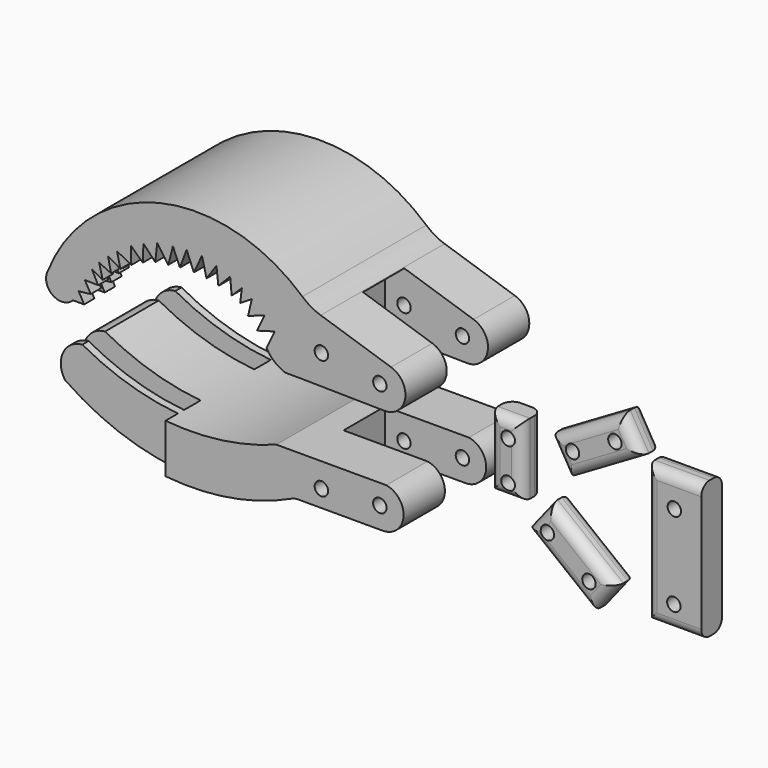
from build123d import *

# Parameters (mm, degrees)
F2_DEPTH       = 38.1
F3_DEPTH       = 38.1
F1_W           = 6.35
F1_H           = 59.9533222238
F4_DEPTH       = 50.8
F1_W_2         = 38.1
F7_DEPTH       = 101.6
F11_D          = 6.604
F11_2_D        = 6.604
F12_W          = 25.4
F12_H          = 93.7925264519
F13_DEPTH      = 25.4
F16_D          = 6.604
F16_DEPTH      = 38.101
F16_2_D        = 6.604
F16_2_DEPTH    = 38.101
F17_D          = 6.604
F17_2_D        = 6.604
F18_W          = 7.62
F18_H          = 40.64
F19_DEPTH      = 76.2
F18_W_2        = 10.16
F0_W           = 15.8650130033
F0_H           = 34.8350182176
F22_DEPTH      = 12.7
F0_W_2         = 26.9726514816
F0_H_2         = 67.5600729883
F23_D          = 6.604
F23_2_D        = 6.604
F23_3_D        = 6.604
F23_4_D        = 6.604
F24_T1_DEPTH   = 60.2350182176
F24_T3_DEPTH   = 41.2650130033
F24_2_T1_DEPTH = 43.5777924299
F24_2_T3_DEPTH = 43.5777924299
F24_2_T5_DEPTH = 66.6787329406
F24_2_T7_DEPTH = 66.6787329406
F24_3_T1_DEPTH = 52.3726514816
F24_3_T3_DEPTH = 92.9600729883
F24_4_T1_DEPTH = 66.6787329406
F24_4_T3_DEPTH = 66.6787329406
F24_4_T5_DEPTH = 43.5777924299
F24_4_T7_DEPTH = 43.5777924299


# Not quite as in the source:
# - a fillet or chamfer that OpenCascade refuses, or shapes differently, is made with other operations: its cross-section is extruded or revolved along the edge and cut away or added


with BuildPart() as f2:
    # F0 (on Front) → F2 (new body, symmetric)
    with BuildSketch(Plane.XZ):
        with BuildLine():
            ThreePointArc((-128.8251806366, 24.5439261482), (-120.2352063415, 28.3244505451), (-114.4677234787, 20.9206566167))
            ThreePointArc((-114.4677234787, 20.9206566167), (-115.0121445518, 18.0890647902), (-116.567776135, 15.6612433482))
            Line((-116.567776135, 15.6612433482), (-111.0370755196, 15.6612433482))
            Line((-111.0370755196, 15.6612433482), (-113.6851459746, 20.5360539255))
            Line((-113.6851459746, 20.5360539255), (-107.745103538, 21.214004606))
            Line((-107.745103538, 21.214004606), (-110.6837838888, 26.4116507024))
            Line((-110.6837838888, 26.4116507024), (-104.1332259774, 26.230096817))
            Line((-104.1332259774, 26.230096817), (-107.1282997727, 32.1294739842))
            Line((-107.1282997727, 32.1294739842), (-101.9096150994, 29.2251650244))
            Line((-101.9096150994, 29.2251650244), (-103.6340519786, 36.2136624753))
            Line((-103.6340519786, 36.2136624753), (-97.7411866188, 33.430468291))
            Line((-97.7411866188, 33.430468291), (-99.2413535714, 40.3858050704))
            Line((-99.2413535714, 40.3858050704), (-93.1724831462, 36.8399471045))
            Line((-93.1724831462, 36.8399471045), (-94.8431268334, 44.0680421889))
            Line((-94.8431268334, 44.0680421889), (-87.853692472, 40.2494259179))
            Line((-87.853692472, 40.2494259179), (-87.853692472, 48.4662689269))
            Line((-87.853692472, 48.4662689269), (-82.1257680654, 43.1474819779))
            Line((-82.1257680654, 43.1474819779), (-81.8530097604, 51.6029894352))
            Line((-81.8530097604, 51.6029894352), (-76.0227963328, 45.3636422753))
            Line((-76.0227963328, 45.3636422753), (-75.0340521335, 53.9896264672))
            Line((-75.0340521335, 53.9896264672), (-69.6129798889, 46.2842024863))
            Line((-69.6129798889, 46.2842024863), (-67.3286244273, 55.1488474011))
            Line((-67.3286244273, 55.1488474011), (-63.8850554824, 46.9320043921))
            Line((-63.8850554824, 46.9320043921), (-60.5778545141, 55.8307431638))
            Line((-60.5778545141, 55.8307431638), (-57.0319965482, 47.0683835447))
            Line((-57.0319965482, 47.0683835447), (-53.008813411, 55.6943640113))
            Line((-53.008813411, 55.6943640113), (-50.7926493883, 46.5228669345))
            Line((-50.7926493883, 46.5228669345), (-45.9170974791, 53.6486767232))
            Line((-45.9170974791, 53.6486767232), (-44.9624434113, 45.1590754092))
            Line((-44.9624434113, 45.1590754092), (-39.1663275659, 51.1597581208))
            Line((-39.1663275659, 51.1597581208), (-38.4162440896, 43.1474819779))
            Line((-38.4162440896, 43.1474819779), (-33.4043093026, 47.9889400303))
            Line((-33.4043093026, 47.9889400303), (-34.2225842178, 41.2722676992))
            Line((-34.2225842178, 41.2722676992), (-28.4946598112, 44.8181256652))
            Line((-28.4946598112, 44.8181256652), (-30.3357802331, 36.9081310928))
            Line((-30.3357802331, 36.9081310928), (-22.2009439021, 39.8494154215))
            Line((-22.2009439021, 39.8494154215), (-26.0398332029, 31.9643877447))
            Line((-26.0398332029, 31.9643877447), (-17.2234997153, 34.4656482339))
            Line((-17.2234997153, 34.4656482339), (-21.2665628641, 25.99779889))
            ThreePointArc((-21.2665628641, 25.99779889), (-17.3327439292, 21.2846448873), (-11.9722324247, 18.2923767716))
            Line((-11.9722324247, 18.2923767716), (-5.0168965772, 18.2923767716))
            Line((-5.0168965772, 18.2923767716), (36.7117887588, 17.6685203985))
            ThreePointArc((36.7117887588, 17.6685203985), (26.7700458222, 29.5718005255), (40.0189591139, 37.6336010062))
            Line((40.0189591139, 37.6336010062), (5.4235169889, 48.8439725139))
            ThreePointArc((5.4235169889, 48.8439725139), (0.643395485, 50.9582523352), (-3.6027484392, 54.0062028812))
            ThreePointArc((-3.6027484392, 54.0062028812), (-73.8525944836, 71.7412526891), (-128.8251806366, 24.5439261482))
        make_face()
        with BuildLine():
            ThreePointArc((-116.567776135, 15.6612433482), (-115.0121445518, 18.0890647902), (-114.4677234787, 20.9206566167))
            ThreePointArc((-114.4677234787, 20.9206566167), (-120.2352063415, 28.3244505451), (-128.8251806366, 24.5439261482))
            ThreePointArc((-128.8251806366, 24.5439261482), (-129.0377711486, 17.7229988191), (-123.7120369893, 13.4560561175))
            ThreePointArc((-123.7120369893, 13.4560561175), (-119.8571320545, 13.6226834922), (-116.5758461433, 15.6527621871))
            Line((-116.5758461433, 15.6527621871), (-116.5844935908, 15.6612433482))
            Line((-116.5844935908, 15.6612433482), (-116.567776135, 15.6612433482))
        make_face()
        with BuildLine():
            ThreePointArc((47.0970060859, 27.8996361516), (45.1404294961, 33.9172939337), (40.0189591139, 37.6336010062))
            ThreePointArc((40.0189591139, 37.6336010062), (26.7700458222, 29.5718005255), (36.7117887588, 17.6685203985))
            ThreePointArc((36.7117887588, 17.6685203985), (44.0457642548, 20.610458069), (47.0970060859, 27.8996361516))
        make_face()
    extrude(amount=F2_DEPTH, both=True)


with BuildPart() as f3:
    # F0 (on Front) → F3 (new body, symmetric)
    with BuildSketch(Plane.XZ):
        with BuildLine():
            ThreePointArc((-16.3927662015, -14.2879039049), (-67.9891228697, -21.918815215), (-117.9927662015, -7.0847165771))
            ThreePointArc((-117.9927662015, -7.0847165771), (-127.4987000517, -13.6840940744), (-126.5054345131, -25.2135340124))
            ThreePointArc((-126.5054345131, -25.2135340124), (-68.9044594779, -45.9426399436), (-8.6425119871, -35.1692541094))
            ThreePointArc((-8.6425119871, -35.1692541094), (-7.3286334335, -34.7213280214), (-5.9488167833, -34.5696024597))
            Line((-5.9488167833, -34.5696024597), (35.9885878861, -34.5696024597))
            ThreePointArc((35.9885878861, -34.5696024597), (46.1644449099, -25.2048799221), (37.6752912998, -14.2879039049))
            Line((37.6752912998, -14.2879039049), (-16.3927662015, -14.2879039049))
        make_face()
    extrude(amount=F3_DEPTH, both=True)


with BuildPart() as f4:
    # F1 (on Right) → F4 (new body, symmetric)
    with BuildSketch(Plane.YZ):
        with Locations((-28.575, 0)):
            Rectangle(F1_W, F1_H)
    extrude(amount=F4_DEPTH, both=True)


with BuildPart() as f4b:
    # F1 (on Right) → F4, piece 2 (new body, symmetric)
    with BuildSketch(Plane.YZ):
        with Locations((28.575, 0)):
            Rectangle(F1_W, F1_H)
    extrude(amount=F4_DEPTH, both=True)


with BuildPart() as f4c:
    # F1 (on Right) → F4, piece 3 (new body, symmetric)
    with BuildSketch(Plane.YZ):
        Rectangle(F1_W_2, F1_H)
    extrude(amount=F4_DEPTH, both=True)


with BuildPart() as f4b_1:
    # F5: moved
    add(f4b.part.moved(Location((-127.83619, 0, 26.70263))))


with BuildPart() as f4c_1:
    # F5: moved
    add(f4c.part.moved(Location((-127.83619, 0, 26.70263))))


with BuildPart() as f4_1:
    # F5: moved
    add(f4.part.moved(Location((-127.83619, 0, 26.70263))))


with BuildPart() as f2_1:
    add(f2.part)

    # F6: cut F4b, F4c, F4
    add(f4b_1.part, mode=Mode.SUBTRACT)
    add(f4c_1.part, mode=Mode.SUBTRACT)
    add(f4_1.part, mode=Mode.SUBTRACT)

    # F11 (through all)
    with Locations(Plane.XZ.offset(38.1)):
        with Locations((34.5100872219, 28.6537986249), (34.5100872219, -24.0924805403)):
            Hole(F11_D / 2)


with BuildPart() as f7:
    # F1 (on Right) → F7 (new body)
    with BuildSketch(Plane.YZ):
        with Locations((34.925, 0)):
            Rectangle(F1_W, F1_H)
    extrude(amount=F7_DEPTH)


with BuildPart() as f7b:
    # F1 (on Right) → F7, piece 2 (new body)
    with BuildSketch(Plane.YZ):
        with Locations((22.225, 0)):
            Rectangle(F1_W, F1_H)
    extrude(amount=F7_DEPTH)


with BuildPart() as f7c:
    # F1 (on Right) → F7, piece 3 (new body)
    with BuildSketch(Plane.YZ):
        with Locations((-22.225, 0)):
            Rectangle(F1_W, F1_H)
    extrude(amount=F7_DEPTH)


with BuildPart() as f7d:
    # F1 (on Right) → F7, piece 4 (new body)
    with BuildSketch(Plane.YZ):
        with Locations((-34.925, 0)):
            Rectangle(F1_W, F1_H)
    extrude(amount=F7_DEPTH)


with BuildPart() as f7d_1:
    # F8: moved
    add(f7d.part.moved(Location((-172.56578, 0, -27.78))))


with BuildPart() as f7c_1:
    # F8: moved
    add(f7c.part.moved(Location((-172.56578, 0, -27.78))))


with BuildPart() as f7_1:
    # F8: moved
    add(f7.part.moved(Location((-172.56578, 0, -27.78))))


with BuildPart() as f7b_1:
    # F8: moved
    add(f7b.part.moved(Location((-172.56578, 0, -27.78))))


with BuildPart() as f3_1:
    add(f3.part)

    # F9: cut F7, F7b, F7c, F7d
    add(f7_1.part, mode=Mode.SUBTRACT)
    add(f7b_1.part, mode=Mode.SUBTRACT)
    add(f7c_1.part, mode=Mode.SUBTRACT)
    add(f7d_1.part, mode=Mode.SUBTRACT)

    # F11#2 (through all)
    with Locations(Plane.XZ.offset(38.1)):
        with Locations((34.5100872219, 28.6537986249), (34.5100872219, -24.0924805403)):
            Hole(F11_2_D / 2)


with BuildPart() as f13:
    # F12 (on Right) → F13 (new body, symmetric)
    with BuildSketch(Plane.YZ):
        Rectangle(F12_W, F12_H)
    extrude(amount=F13_DEPTH, both=True)


with BuildPart() as f13_1:
    # F14: moved
    add(f13.part.moved(Location((21.74683, 0, 1.79154))))


with BuildPart() as f2_2:
    add(f2_1.part)

    # F15: cut F13
    add(f13_1.part, mode=Mode.SUBTRACT)

    # F16 (through all, one way)
    with BuildSketch(Plane(origin=(0, 0, 0), x_dir=(1, 0, 0), z_dir=(0, 1, 0))):
        with Locations((5.7323579676, -32.5988233089), (5.7323579676, 26.1833130696)):
            Circle(F16_D / 2)
    extrude(amount=-F16_DEPTH, mode=Mode.SUBTRACT)

    # F17 (through all)
    with Locations(Plane.XZ):
        with Locations((5.7323579676, 32.5988233089), (5.7323579676, -26.1833130696)):
            Hole(F17_D / 2)


with BuildPart() as f3_2:
    add(f3_1.part)

    # F15: cut F13
    add(f13_1.part, mode=Mode.SUBTRACT)

    # F16#2 (through all, one way)
    with BuildSketch(Plane(origin=(0, 0, 0), x_dir=(1, 0, 0), z_dir=(0, 1, 0))):
        with Locations((5.7323579676, -32.5988233089), (5.7323579676, 26.1833130696)):
            Circle(F16_2_D / 2)
    extrude(amount=-F16_2_DEPTH, mode=Mode.SUBTRACT)

    # F17#2 (through all)
    with Locations(Plane.XZ):
        with Locations((5.7323579676, 32.5988233089), (5.7323579676, -26.1833130696)):
            Hole(F17_2_D / 2)


with BuildPart() as f19:
    # F18 (on Right) → F19 (new body)
    with BuildSketch(Plane.YZ):
        with Locations((-34.2883425851, -25.9859772711)):
            Rectangle(F18_W, F18_H)
    extrude(amount=F19_DEPTH)


with BuildPart() as f19b:
    # F18 (on Right) → F19, piece 2 (new body)
    with BuildSketch(Plane.YZ):
        with Locations((-21.5883425851, -25.9859772711)):
            Rectangle(F18_W_2, F18_H)
    extrude(amount=F19_DEPTH)


with BuildPart() as f19c:
    # F18 (on Right) → F19, piece 3 (new body)
    with BuildSketch(Plane.YZ):
        with Locations((21.5916574149, -25.9859772711)):
            Rectangle(F18_W_2, F18_H)
    extrude(amount=F19_DEPTH)


with BuildPart() as f19d:
    # F18 (on Right) → F19, piece 4 (new body)
    with BuildSketch(Plane.YZ):
        with Locations((34.2916574149, -25.9859772711)):
            Rectangle(F18_W, F18_H)
    extrude(amount=F19_DEPTH)


with BuildPart() as f19b_1:
    # F20: moved
    add(f19b.part.moved(Location((-147.20744, 0, 0))))


with BuildPart() as f19c_1:
    # F20: moved
    add(f19c.part.moved(Location((-147.20744, 0, 0))))


with BuildPart() as f19d_1:
    # F20: moved
    add(f19d.part.moved(Location((-147.20744, 0, 0))))


with BuildPart() as f19_1:
    # F20: moved
    add(f19.part.moved(Location((-147.20744, 0, 0))))


with BuildPart() as f3_3:
    add(f3_2.part)

    # F21: cut F19d, F19c, F19b, F19
    add(f19d_1.part, mode=Mode.SUBTRACT)
    add(f19c_1.part, mode=Mode.SUBTRACT)
    add(f19b_1.part, mode=Mode.SUBTRACT)
    add(f19_1.part, mode=Mode.SUBTRACT)


with BuildPart() as f22:
    # F0 (on Front) → F22 (new body)
    with BuildSketch(Plane.XZ):
        with Locations((76.168358326, 0)):
            Rectangle(F0_W, F0_H)
    extrude(amount=F22_DEPTH)

    # F23 (through all)
    with Locations(Plane(origin=(0, 0, 0), x_dir=(1, 0, 0), z_dir=(0, 1, 0))):
        with Locations((77.2331506014, -8.5078338161), (77.2331506014, 10.8820619062), (108.9814379811, -13.1955016404), (129.8628747463, -24.2754425853), (96.6230481863, 26.0104443878), (117.0783191919, 40.4995940626), (159.1015905142, -4.5702983625), (158.8720083237, 36.766640842)):
            Hole(F23_D / 2)

    # F24: fillet of radius 5.08 on 7 edges, made by hand

    # F24_s2 → F24_t1 (cut)
    with BuildSketch(Plane.XY.offset(-30.1175091088)):
        with BuildLine():
            ThreePointArc((84.1008648276, -5.08), (82.6129672761, -1.4878975516), (79.0208648276, 0))
            Line((79.0208648276, 0), (84.1008648276, 0))
            Line((84.1008648276, 0), (84.1008648276, -5.08))
        make_face()
        with BuildLine():
            ThreePointArc((68.2358518243, -5.08), (69.7237493759, -1.4878975516), (73.3158518243, 0))
            Line((73.3158518243, 0), (68.2358518243, 0))
            Line((68.2358518243, 0), (68.2358518243, -5.08))
        make_face()
        with BuildLine():
            ThreePointArc((84.1008648276, -7.62), (82.6129672761, -11.2121024484), (79.0208648276, -12.7))
            Line((79.0208648276, -12.7), (84.1008648276, -12.7))
            Line((84.1008648276, -12.7), (84.1008648276, -7.62))
        make_face()
        with BuildLine():
            ThreePointArc((68.2358518243, -7.62), (69.7237493759, -11.2121024484), (73.3158518243, -12.7))
            Line((73.3158518243, -12.7), (68.2358518243, -12.7))
            Line((68.2358518243, -12.7), (68.2358518243, -7.62))
        make_face()
    extrude(amount=F24_T1_DEPTH, mode=Mode.SUBTRACT)

    # F24_s4 → F24_t3 (cut)
    with BuildSketch(Plane.YZ.offset(55.5358518243)):
        with BuildLine():
            ThreePointArc((-5.08, -17.4175091088), (-1.4878975516, -15.9296115572), (0, -12.3375091088))
            Line((0, -12.3375091088), (0, -17.4175091088))
            Line((0, -17.4175091088), (-5.08, -17.4175091088))
        make_face()
        with BuildLine():
            ThreePointArc((-7.62, -17.4175091088), (-11.2121024484, -15.9296115572), (-12.7, -12.3375091088))
            Line((-12.7, -12.3375091088), (-12.7, -17.4175091088))
            Line((-12.7, -17.4175091088), (-7.62, -17.4175091088))
        make_face()
        with BuildLine():
            ThreePointArc((-12.7, 12.3375091088), (-11.2121024484, 15.9296115572), (-7.62, 17.4175091088))
            Line((-7.62, 17.4175091088), (-12.7, 17.4175091088))
            Line((-12.7, 17.4175091088), (-12.7, 12.3375091088))
        make_face()
    extrude(amount=F24_T3_DEPTH, mode=Mode.SUBTRACT)


with BuildPart() as f22b:
    # F0 (on Front) → F22, piece 2 (new body)
    with BuildSketch(Plane.XZ):
        Polygon((142.5378596938, 21.2889943894), (133.362479084, 36.9811748718), (97.7281560559, 16.1454167741), (106.9035366657, 0.4532362917), align=None)
    extrude(amount=F22_DEPTH)

    # F23#2 (through all)
    with Locations(Plane(origin=(0, 0, 0), x_dir=(1, 0, 0), z_dir=(0, 1, 0))):
        with Locations((77.2331506014, -8.5078338161), (77.2331506014, 10.8820619062), (108.9814379811, -13.1955016404), (129.8628747463, -24.2754425853), (96.6230481863, 26.0104443878), (117.0783191919, 40.4995940626), (159.1015905142, -4.5702983625), (158.8720083237, 36.766640842)):
            Hole(F23_2_D / 2)

    # F24#2: fillet of radius 5.08 on 8 edges, made by hand

    # F24_2_s2 → F24_2_t1 (cut)
    with BuildSketch(Plane(origin=(11.4536229743, 0, -19.588540959), x_dir=(0, 1, 0), z_dir=(0.5047576951, 0, -0.8632610666))):
        with BuildLine():
            ThreePointArc((-7.62, 92.5144355963), (-11.2121024484, 94.0023331479), (-12.7, 97.5944355963))
            Line((-12.7, 97.5944355963), (-12.7, 92.5144355963))
            Line((-12.7, 92.5144355963), (-7.62, 92.5144355963))
        make_face()
        with BuildLine():
            ThreePointArc((-5.08, 92.5144355963), (-1.4878975516, 94.0023331479), (0, 97.5944355963))
            Line((0, 97.5944355963), (0, 92.5144355963))
            Line((0, 92.5144355963), (-5.08, 92.5144355963))
        make_face()
    extrude(amount=F24_2_T1_DEPTH, mode=Mode.SUBTRACT)

    # F24_2_s4 → F24_2_t3 (cut)
    with BuildSketch(Plane(origin=(33.4498490409, 0, -57.2075525342), x_dir=(0, 1, 0), z_dir=(-0.5047576951, 0, 0.8632610666))):
        with BuildLine():
            ThreePointArc((-7.62, -133.7931685369), (-11.2121024484, -132.3052709853), (-12.7, -128.7131685369))
            Line((-12.7, -128.7131685369), (-12.7, -133.7931685369))
            Line((-12.7, -133.7931685369), (-7.62, -133.7931685369))
        make_face()
        with BuildLine():
            ThreePointArc((-5.08, -133.7931685369), (-1.4878975516, -132.3052709853), (0, -128.7131685369))
            Line((0, -128.7131685369), (0, -133.7931685369))
            Line((0, -133.7931685369), (-5.08, -133.7931685369))
        make_face()
    extrude(amount=F24_2_T3_DEPTH, mode=Mode.SUBTRACT)

    # F24_2_s6 → F24_2_t5 (cut)
    with BuildSketch(Plane(origin=(68.9006948068, 0, 40.2869505511), x_dir=(0, 1, 0), z_dir=(0.8632610666, 0, 0.5047576951))):
        with BuildLine():
            ThreePointArc((-12.7, -48.4891215259), (-11.2121024484, -52.0812239743), (-7.62, -53.5691215259))
            Line((-7.62, -53.5691215259), (-12.7, -53.5691215259))
            Line((-12.7, -53.5691215259), (-12.7, -48.4891215259))
        make_face()
        with BuildLine():
            ThreePointArc((0, -48.4891215259), (-1.4878975516, -52.0812239743), (-5.08, -53.5691215259))
            Line((-5.08, -53.5691215259), (0, -53.5691215259))
            Line((0, -53.5691215259), (0, -48.4891215259))
        make_face()
    extrude(amount=F24_2_T5_DEPTH, mode=Mode.SUBTRACT)

    # F24_2_s8 → F24_2_t7 (cut)
    with BuildSketch(Plane(origin=(126.4618489277, 0, 73.9435541056), x_dir=(0, 1, 0), z_dir=(-0.8632610666, 0, -0.5047576951))):
        with BuildLine():
            ThreePointArc((-7.62, 35.3913290959), (-11.2121024484, 36.8792266475), (-12.7, 40.4713290959))
            Line((-12.7, 40.4713290959), (-12.7, 35.3913290959))
            Line((-12.7, 35.3913290959), (-7.62, 35.3913290959))
        make_face()
        with BuildLine():
            ThreePointArc((-5.08, 35.3913290959), (-1.4878975516, 36.8792266475), (0, 40.4713290959))
            Line((0, 40.4713290959), (0, 35.3913290959))
            Line((0, 35.3913290959), (-5.08, 35.3913290959))
        make_face()
    extrude(amount=F24_2_T7_DEPTH, mode=Mode.SUBTRACT)


with BuildPart() as f22c:
    # F0 (on Front) → F22, piece 3 (new body)
    with BuildSketch(Plane.XZ):
        with Locations((158.8787287474, -14.537781477)):
            Rectangle(F0_W_2, F0_H_2)
    extrude(amount=F22_DEPTH)

    # F23#3 (through all)
    with Locations(Plane(origin=(0, 0, 0), x_dir=(1, 0, 0), z_dir=(0, 1, 0))):
        with Locations((77.2331506014, -8.5078338161), (77.2331506014, 10.8820619062), (108.9814379811, -13.1955016404), (129.8628747463, -24.2754425853), (96.6230481863, 26.0104443878), (117.0783191919, 40.4995940626), (159.1015905142, -4.5702983625), (158.8720083237, 36.766640842)):
            Hole(F23_3_D / 2)

    # F24#3: fillet of radius 5.08 on 6 edges, made by hand

    # F24_3_s2 → F24_3_t1 (cut)
    with BuildSketch(Plane.YZ.offset(132.6924030066)):
        with BuildLine():
            ThreePointArc((-7.62, -48.3178179711), (-11.2121024484, -46.8299204195), (-12.7, -43.2378179711))
            Line((-12.7, -43.2378179711), (-12.7, -48.3178179711))
            Line((-12.7, -48.3178179711), (-7.62, -48.3178179711))
        make_face()
        with BuildLine():
            ThreePointArc((-5.08, -48.3178179711), (-1.4878975516, -46.8299204195), (0, -43.2378179711))
            Line((0, -43.2378179711), (0, -48.3178179711))
            Line((0, -48.3178179711), (-5.08, -48.3178179711))
        make_face()
        with BuildLine():
            ThreePointArc((-7.62, 19.2422550172), (-11.2121024484, 17.7543574656), (-12.7, 14.1622550172))
            Line((-12.7, 14.1622550172), (-12.7, 19.2422550172))
            Line((-12.7, 19.2422550172), (-7.62, 19.2422550172))
        make_face()
        with BuildLine():
            ThreePointArc((-5.08, 19.2422550172), (-1.4878975516, 17.7543574656), (0, 14.1622550172))
            Line((0, 14.1622550172), (0, 19.2422550172))
            Line((0, 19.2422550172), (-5.08, 19.2422550172))
        make_face()
    extrude(amount=F24_3_T1_DEPTH, mode=Mode.SUBTRACT)

    # F24_3_s4 → F24_3_t3 (cut)
    with BuildSketch(Plane.XY.offset(-61.0178179711)):
        with BuildLine():
            ThreePointArc((150.4724030066, -12.7), (146.8803005581, -11.2121024484), (145.3924030066, -7.62))
            Line((145.3924030066, -7.62), (145.3924030066, -12.7))
            Line((145.3924030066, -12.7), (150.4724030066, -12.7))
        make_face()
        with BuildLine():
            ThreePointArc((150.4724030066, 0), (146.8803005581, -1.4878975516), (145.3924030066, -5.08))
            Line((145.3924030066, -5.08), (145.3924030066, 0))
            Line((145.3924030066, 0), (150.4724030066, 0))
        make_face()
    extrude(amount=F24_3_T3_DEPTH, mode=Mode.SUBTRACT)


with BuildPart() as f22d:
    # F0 (on Front) → F22, piece 4 (new body)
    with BuildSketch(Plane.XZ):
        Polygon((86.3592635802, -27.7551872225), (118.7411078658, -53.3549910077), (130.0144170569, -39.0950948823), (97.6325727713, -13.495291097), align=None)
    extrude(amount=F22_DEPTH)

    # F23#4 (through all)
    with Locations(Plane(origin=(0, 0, 0), x_dir=(1, 0, 0), z_dir=(0, 1, 0))):
        with Locations((77.2331506014, -8.5078338161), (77.2331506014, 10.8820619062), (108.9814379811, -13.1955016404), (129.8628747463, -24.2754425853), (96.6230481863, 26.0104443878), (117.0783191919, 40.4995940626), (159.1015905142, -4.5702983625), (158.8720083237, 36.766640842)):
            Hole(F23_4_D / 2)

    # F24#4: fillet of radius 5.08 on 8 edges, made by hand

    # F24_4_s2 → F24_4_t1 (cut)
    with BuildSketch(Plane(origin=(108.9921971516, 0, -86.1649150247), x_dir=(0, 1, 0), z_dir=(-0.7844679809, 0, 0.6201693211))):
        with BuildLine():
            ThreePointArc((-7.62, -49.9621026177), (-11.2121024484, -48.4742050661), (-12.7, -44.8821026177))
            Line((-12.7, -44.8821026177), (-12.7, -49.9621026177))
            Line((-12.7, -49.9621026177), (-7.62, -49.9621026177))
        make_face()
        with BuildLine():
            ThreePointArc((-5.08, -49.9621026177), (-1.4878975516, -48.4742050661), (0, -44.8821026177))
            Line((0, -44.8821026177), (0, -49.9621026177))
            Line((0, -49.9621026177), (-5.08, -49.9621026177))
        make_face()
    extrude(amount=F24_4_T1_DEPTH, mode=Mode.SUBTRACT)

    # F24_4_s4 → F24_4_t3 (cut)
    with BuildSketch(Plane(origin=(56.6848661503, 0, -44.8128104825), x_dir=(0, 1, 0), z_dir=(0.7844679809, 0, -0.6201693211))):
        with BuildLine():
            ThreePointArc((-12.7, 36.8643101878), (-11.2121024484, 33.2722077393), (-7.62, 31.7843101878))
            Line((-7.62, 31.7843101878), (-12.7, 31.7843101878))
            Line((-12.7, 31.7843101878), (-12.7, 36.8643101878))
        make_face()
        with BuildLine():
            ThreePointArc((0, 36.8643101878), (-1.4878975516, 33.2722077393), (-5.08, 31.7843101878))
            Line((-5.08, 31.7843101878), (0, 31.7843101878))
            Line((0, 31.7843101878), (0, 36.8643101878))
        make_face()
    extrude(amount=F24_4_T3_DEPTH, mode=Mode.SUBTRACT)

    # F24_4_s6 → F24_4_t5 (cut)
    with BuildSketch(Plane(origin=(11.8355036936, 0, 14.9710302806), x_dir=(0, 1, 0), z_dir=(0.6201693211, 0, 0.7844679809))):
        with BuildLine():
            ThreePointArc((-7.62, -126.2377256945), (-11.2121024484, -124.7498281429), (-12.7, -121.1577256945))
            Line((-12.7, -121.1577256945), (-12.7, -126.2377256945))
            Line((-12.7, -126.2377256945), (-7.62, -126.2377256945))
        make_face()
        with BuildLine():
            ThreePointArc((-5.08, -126.2377256945), (-1.4878975516, -124.7498281429), (0, -121.1577256945))
            Line((0, -121.1577256945), (0, -126.2377256945))
            Line((0, -126.2377256945), (-5.08, -126.2377256945))
        make_face()
    extrude(amount=F24_4_T5_DEPTH, mode=Mode.SUBTRACT)

    # F24_4_s8 → F24_4_t7 (cut)
    with BuildSketch(Plane(origin=(38.8611136416, 0, 49.1564131218), x_dir=(0, 1, 0), z_dir=(-0.6201693211, 0, -0.7844679809))):
        with BuildLine():
            ThreePointArc((-7.62, 84.9589927539), (-11.2121024484, 86.4468903055), (-12.7, 90.0389927539))
            Line((-12.7, 90.0389927539), (-12.7, 84.9589927539))
            Line((-12.7, 84.9589927539), (-7.62, 84.9589927539))
        make_face()
        with BuildLine():
            ThreePointArc((-5.08, 84.9589927539), (-1.4878975516, 86.4468903055), (0, 90.0389927539))
            Line((0, 90.0389927539), (0, 84.9589927539))
            Line((0, 84.9589927539), (-5.08, 84.9589927539))
        make_face()
    extrude(amount=F24_4_T7_DEPTH, mode=Mode.SUBTRACT)


solid = Compound([f2_2.part, f3_3.part, f22.part, f22b.part, f22c.part, f22d.part])
